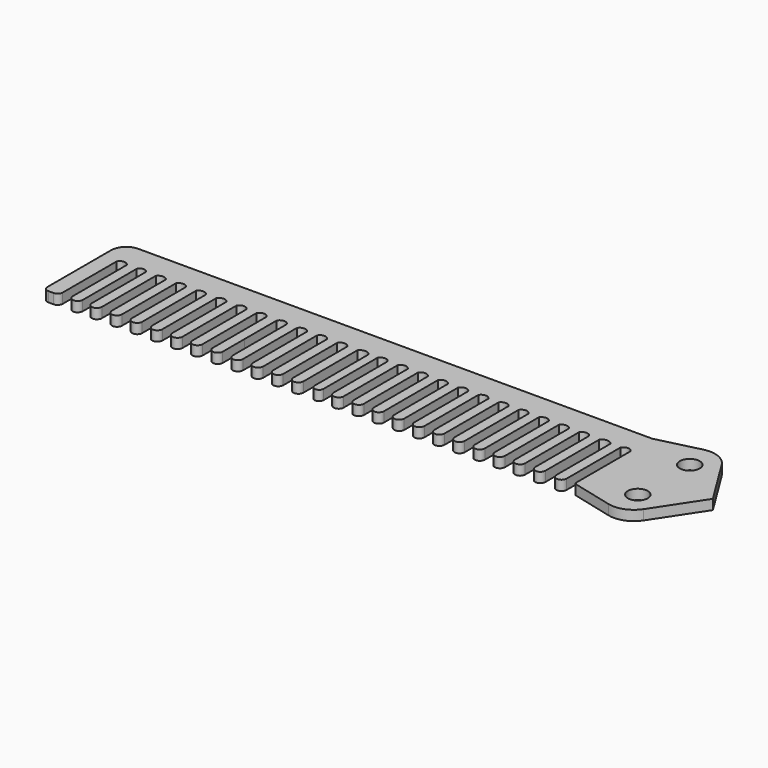
from build123d import *

# Parameters (mm, degrees)
F0_R     = 2
F1_DEPTH = 2


# Not quite as in the source:
# - a feature names something its author has since deleted; it is built from what else it names


with BuildPart() as f1:
    # F0 (on Top) → F1 (new body)
    with BuildSketch(Plane.XY):
        with BuildLine():
            ThreePointArc((-47.5321587284, -3.0349094544), (-47.2359537694, -3.7500114836), (-46.5208517402, -4.0462164426))
            Line((-46.5208517402, -4.0462164426), (-45.4874065769, -4.0462164426))
            ThreePointArc((-45.4874065769, -4.0462164426), (-44.7723045476, -3.7500114836), (-44.4760995886, -3.0349094544))
            Line((-44.4760995886, -3.0349094544), (-44.4760995886, 10.5057977874))
            ThreePointArc((-44.4760995886, 10.5057977874), (-43.4758616879, 11.1175826134), (-42.4756237872, 10.5057977874))
            Line((-42.4756237872, 10.5057977874), (-42.4756237872, -3.0349094544))
            Line((-42.4756237872, -3.0349094544), (-42.4756237872, -3.0449686175))
            ThreePointArc((-42.4756237872, -3.0449686175), (-41.464329306, -4.0512460242), (-40.4530348247, -3.0449686175))
            Line((-40.4530348247, -3.0449686175), (-40.4530348247, -3.0349094544))
            Line((-40.4530348247, -3.0349094544), (-40.4530348247, 2.3688513962))
            Line((-40.4530348247, 2.3688513962), (-40.4530348247, 10.5057977874))
            ThreePointArc((-40.4530348247, 10.5057977874), (-39.5547852119, 11.0928656343), (-38.6565355991, 10.5057977874))
            Line((-38.6565355991, 10.5057977874), (-38.6565355991, 2.3688513962))
            Line((-38.6565355991, 2.3688513962), (-38.6565355991, -3.0349094544))
            ThreePointArc((-38.6565355991, -3.0349094544), (-37.6453452622, -4.0308565278), (-36.6341549253, -3.0349094544))
            Line((-36.6341549253, -3.0349094544), (-36.6341549253, 2.3688513962))
            Line((-36.6341549253, 2.3688513962), (-36.6341549253, 10.5057977874))
            ThreePointArc((-36.6341549253, 10.5057977874), (-35.6227312857, 11.0363635), (-34.6113076461, 10.5057977874))
            Line((-34.6113076461, 10.5057977874), (-34.6113076461, 2.3688513962))
            Line((-34.6113076461, 2.3688513962), (-34.6113076461, -3.0349094544))
            ThreePointArc((-34.6113076461, -3.0349094544), (-33.6001581891, -4.0283670709), (-32.5890087321, -3.0349094544))
            Line((-32.5890087321, -3.0349094544), (-32.5890087321, 2.3688513962))
            Line((-32.5890087321, 2.3688513962), (-32.5890087321, 10.5057977874))
            ThreePointArc((-32.5890087321, 10.5057977874), (-31.5775442126, 11.0839798549), (-30.5660796932, 10.5057977874))
            Line((-30.5660796932, 10.5057977874), (-30.5660796932, 2.3688513962))
            Line((-30.5660796932, 2.3688513962), (-30.5660796932, -3.0349094544))
            ThreePointArc((-30.5660796932, -3.0349094544), (-29.5547727049, -4.0320483822), (-28.5434657167, -3.0349094544))
            Line((-28.5434657167, -3.0349094544), (-28.5434657167, 2.3688513962))
            Line((-28.5434657167, 2.3688513962), (-28.5434657167, 10.5057977874))
            ThreePointArc((-28.5434657167, 10.5057977874), (-27.5321587284, 11.0375669764), (-26.5208517402, 10.5057977874))
            Line((-26.5208517402, 10.5057977874), (-26.5208517402, 2.3688513962))
            Line((-26.5208517402, 2.3688513962), (-26.5208517402, -3.0349094544))
            ThreePointArc((-26.5208517402, -3.0349094544), (-25.5095447519, -4.0289367833), (-24.4982377637, -3.0349094544))
            Line((-24.4982377637, -3.0349094544), (-24.4982377637, 2.3688513962))
            Line((-24.4982377637, 2.3688513962), (-24.4982377637, 10.5057977874))
            ThreePointArc((-24.4982377637, 10.5057977874), (-23.4869307754, 11.0979693494), (-22.4756237872, 10.5057977874))
            Line((-22.4756237872, 10.5057977874), (-22.4756237872, 2.3688513962))
            Line((-22.4756237872, 2.3688513962), (-22.4756237872, -3.0349094544))
            ThreePointArc((-22.4756237872, -3.0349094544), (-21.464316799, -4.0179106089), (-20.4530098107, -3.0349094544))
            Line((-20.4530098107, -3.0349094544), (-20.4530098107, 2.3688513962))
            Line((-20.4530098107, 2.3688513962), (-20.4530098107, 10.5057977874))
            ThreePointArc((-20.4530098107, 10.5057977874), (-19.4417028225, 11.112544636), (-18.4303958342, 10.5057977874))
            Line((-18.4303958342, 10.5057977874), (-18.4303958342, 2.3688513962))
            Line((-18.4303958342, 2.3688513962), (-18.4303958342, -3.0349094544))
            ThreePointArc((-18.4303958342, -3.0349094544), (-17.419088846, -4.0462164426), (-16.4077818577, -3.0349094544))
            Line((-16.4077818577, -3.0349094544), (-16.4077818577, 2.3688513962))
            Line((-16.4077818577, 2.3688513962), (-16.4077818577, 10.5057977874))
            ThreePointArc((-16.4077818577, 10.5057977874), (-15.3964748695, 11.0913376707), (-14.3851678813, 10.5057977874))
            Line((-14.3851678813, 10.5057977874), (-14.3851678812, 2.3688513962))
            Line((-14.3851678812, 2.3688513962), (-14.3851678812, -3.0349094544))
            ThreePointArc((-14.3851678812, -3.0349094544), (-13.373860893, -4.0324857923), (-12.3625539048, -3.0349094544))
            Line((-12.3625539048, -3.0349094544), (-12.3625539048, 2.3688513962))
            Line((-12.3625539047, 2.3688513962), (-12.3625539048, 10.5057977874))
            ThreePointArc((-12.3625539048, 10.5057977874), (-11.3512469165, 11.1038299062), (-10.3399399283, 10.5057977874))
            Line((-10.3399399283, 10.5057977874), (-10.3399399283, 2.3688513962))
            Line((-10.3399399283, 2.3688513962), (-10.3399399283, -3.0349094544))
            ThreePointArc((-10.3399399283, -3.0349094544), (-9.32863294, -4.0336439564), (-8.3173259518, -3.0349094544))
            Line((-8.3173259518, -3.0349094544), (-8.3173259518, 2.3688513962))
            Line((-8.3173259518, 2.3688513962), (-8.3173259518, 10.5057977874))
            ThreePointArc((-8.3173259518, 10.5057977874), (-7.3060189635, 11.1037566218), (-6.2947119753, 10.5057977874))
            Line((-6.2947119753, 10.5057977874), (-6.2947119753, 2.3688513962))
            Line((-6.2947119753, 2.3688513962), (-6.2947119753, -3.0349094544))
            ThreePointArc((-6.2947119753, -3.0349094544), (-5.283404987, -4.0328236585), (-4.2720979988, -3.0349094544))
            Line((-4.2720979988, -3.0349094544), (-4.2720979988, 2.3688513962))
            Line((-4.2720979988, 2.3688513962), (-4.2720979988, 10.5057977874))
            ThreePointArc((-4.2720979988, 10.5057977874), (-3.2607910105, 11.1182503387), (-2.2494840223, 10.5057977874))
            Line((-2.2494840223, 10.5057977874), (-2.2494840223, 2.3688513962))
            Line((-2.2494840223, 2.3688513962), (-2.2494840223, -3.0349094544))
            ThreePointArc((-2.2494840223, -3.0349094544), (-1.2381770341, -4.0279358965), (-0.2268700458, -3.0349094544))
            Line((-0.2268700458, -3.0349094544), (-0.2268700458, 2.3688513962))
            Line((-0.2268700458, 2.3688513962), (-0.2268700458, 10.5057977874))
            ThreePointArc((-0.2268700458, 10.5057977874), (0.7844369424, 11.1117892762), (1.7957439307, 10.5057977874))
            Line((1.7957439307, 10.5057977874), (1.7957439307, 2.3688513962))
            Line((1.7957439307, 2.3688513962), (1.7957439307, -3.0349094544))
            ThreePointArc((1.7957439307, -3.0349094544), (2.8070509189, -4.0231444656), (3.8183579072, -3.0349094544))
            Line((3.8183579072, -3.0349094544), (3.8183579072, 2.3688513962))
            Line((3.8183579072, 2.3688513962), (3.8183579072, 10.5057977874))
            ThreePointArc((3.8183579072, 10.5057977874), (4.9481016159, 11.1006888991), (6.0778453246, 10.5057977874))
            Line((6.0778453246, 10.5057977874), (6.0778453246, 2.3688513962))
            Line((6.0778453246, 2.3688513962), (6.0778453246, -3.0349094544))
            ThreePointArc((6.0778453246, -3.0349094544), (6.9707155924, -3.9277797221), (7.8635858601, -3.0349094544))
            Line((7.8635858601, -3.0349094544), (7.8635858601, 2.3688513962))
            Line((7.8635858601, 2.3688513962), (7.8635858601, 10.5057977874))
            ThreePointArc((7.8635858601, 10.5057977874), (8.8748928484, 11.1003156957), (9.8861998366, 10.5057977874))
            Line((9.8861998366, 10.5057977874), (9.8861998366, 2.3688513962))
            Line((9.8861998366, 2.3688513962), (9.8861998366, -3.0349094544))
            ThreePointArc((9.8861998366, -3.0349094544), (10.8975068249, -4.0462164426), (11.9088138131, -3.0349094544))
            Line((11.9088138131, -3.0349094544), (11.9088138131, 2.3688513962))
            Line((11.9088138131, 2.3688513962), (11.9088138131, 10.5057977874))
            ThreePointArc((11.9088138131, 10.5057977874), (12.9201208014, 11.1003953408), (13.9314277896, 10.5057977874))
            Line((13.9314277896, 10.5057977874), (13.9314277896, 2.3688513962))
            Line((13.9314277896, 2.3688513962), (13.9314277896, -3.0349094544))
            ThreePointArc((13.9314277896, -3.0349094544), (14.9427347779, -4.0462164426), (15.9540417661, -3.0349094544))
            Line((15.9540417661, -3.0349094544), (15.9540417661, 2.3688513962))
            Line((15.9540417661, 2.3688513962), (15.9540417661, 10.5057977874))
            ThreePointArc((15.9540417661, 10.5057977874), (16.9653487543, 11.1012729968), (17.9766557426, 10.5057977874))
            Line((17.9766557426, 10.5057977874), (17.9766557426, -3.0349094544))
            Line((17.9766557426, -3.0349094544), (17.9766557426, -3.0600128507))
            ThreePointArc((17.9766557426, -3.0600128507), (18.987884836, -4.0587681408), (19.9991139294, -3.0600128507))
            Line((19.9991139294, -3.0600128507), (19.9991139294, -3.0349094544))
            Line((19.9991139294, -3.0349094544), (19.9991139294, 2.3688513962))
            Line((19.9991139294, 2.3688513962), (19.9991139294, 10.5057977874))
            ThreePointArc((19.9991139294, 10.5057977874), (21.0104988125, 11.0625593301), (22.0218836956, 10.5057977874))
            Line((22.0218836956, 10.5057977874), (22.0218836956, 2.3688513962))
            Line((22.0218836956, 2.3688513962), (22.0218836956, -3.0349094544))
            ThreePointArc((22.0218836956, -3.0349094544), (23.0331906838, -4.0270898738), (24.0444976721, -3.0349094544))
            Line((24.0444976721, -3.0349094544), (24.0444976721, 2.3688513962))
            Line((24.0444976721, 2.3688513962), (24.0444976721, 10.5057977874))
            ThreePointArc((24.0444976721, 10.5057977874), (25.0558046603, 11.1004906415), (26.0671116486, 10.5057977874))
            Line((26.0671116486, 10.5057977874), (26.0671116486, 2.3688513962))
            Line((26.0671116486, 2.3688513962), (26.0671116486, -3.0349094544))
            ThreePointArc((26.0671116486, -3.0349094544), (27.0784186368, -4.0282444578), (28.089725625, -3.0349094544))
            Line((28.089725625, -3.0349094544), (28.089725625, 2.3688513962))
            Line((28.089725625, 2.3688513962), (28.089725625, 10.5057977874))
            ThreePointArc((28.089725625, 10.5057977874), (29.1010326133, 11.1005861122), (30.1123396015, 10.5057977874))
            Line((30.1123396015, 10.5057977874), (30.1123396015, 2.3688513962))
            Line((30.1123396015, 2.3688513962), (30.1123396015, -3.0349094544))
            ThreePointArc((30.1123396015, -3.0349094544), (31.1236465898, -4.0401241658), (32.134953578, -3.0349094544))
            Line((32.134953578, -3.0349094544), (32.134953578, 2.3688513962))
            Line((32.134953578, 2.3688513962), (32.134953578, 10.5057977874))
            ThreePointArc((32.134953578, 10.5057977874), (33.1462605663, 11.0805944093), (34.1575675545, 10.5057977874))
            Line((34.1575675545, 10.5057977874), (34.1575675545, 2.3688513962))
            Line((34.1575675545, 2.3688513962), (34.1575675545, -3.0349094544))
            ThreePointArc((34.1575675545, -3.0349094544), (35.1688745428, -4.0284589293), (36.180181531, -3.0349094544))
            Line((36.180181531, -3.0349094544), (36.180181531, 2.3688513962))
            Line((36.180181531, 2.3688513962), (36.180181531, 10.5057977874))
            ThreePointArc((36.180181531, 10.5057977874), (37.1914885192, 11.0806196167), (38.2027955075, 10.5057977874))
            Line((38.2027955075, 10.5057977874), (38.2027955075, 2.3688513962))
            Line((38.2027955075, 2.3688513962), (38.2027955075, -3.0349094544))
            ThreePointArc((38.2027955075, -3.0349094544), (39.2141024957, -4.0246480782), (40.225409484, -3.0349094544))
            Line((40.225409484, -3.0349094544), (40.225409484, 2.3688513962))
            Line((40.225409484, 2.3688513962), (40.225409484, 10.5057977874))
            ThreePointArc((40.225409484, 10.5057977874), (41.2367164722, 11.0799992786), (42.2480234605, 10.5057977874))
            Line((42.2480234605, 10.5057977874), (42.2480234605, 2.3688513962))
            Line((42.2480234605, 2.3688513962), (42.2480234605, -3.0349094544))
            ThreePointArc((42.2480234605, -3.0349094544), (43.2593304487, -4.0462164426), (44.270637437, -3.0349094544))
            Line((44.270637437, -3.0349094544), (44.270637437, 2.3688513962))
            Line((44.270637437, 2.3688513962), (44.270637437, 10.5057977874))
            ThreePointArc((44.270637437, 10.5057977874), (45.2819444252, 11.0763000676), (46.2932514135, 10.5057977874))
            Line((46.2932514135, 10.5057977874), (46.2932514135, 2.3688513962))
            Line((46.2932514135, 2.3688513962), (46.2932514135, -3.0349094544))
            ThreePointArc((46.2932514135, -3.0349094544), (47.3045584017, -4.0362897846), (48.3158653899, -3.0349094544))
            Line((48.3158653899, -3.0349094544), (48.3158653899, 2.3688513962))
            Line((48.3158653899, 2.3688513962), (48.3158653899, 10.5057977874))
            ThreePointArc((48.3158653899, 10.5057977874), (49.3271723782, 11.0768378201), (50.3384793664, 10.5057977874))
            Line((50.3384793664, 10.5057977874), (50.3384793664, 2.3688513962))
            Line((50.3384793664, 2.3688513962), (50.3384793664, -3.0349094544))
            ThreePointArc((50.3384793664, -3.0349094544), (51.3497863547, -4.0273604844), (52.3610933429, -3.0349094544))
            Line((52.3610933429, -3.0349094544), (52.3610933429, 2.3688513962))
            Line((52.3610933429, 2.3688513962), (52.3610933429, 10.5057977874))
            ThreePointArc((52.3610933429, 10.5057977874), (53.4851541573, 11.0994017223), (54.6092149717, 10.5057977874))
            Line((54.6092149717, 10.5057977874), (54.6092149717, 2.3688513962))
            Line((54.6092149717, 2.3688513962), (54.6092149717, -3.0349094544))
            ThreePointArc((54.6092149717, -3.0349094544), (55.6205026048, -4.039959639), (56.6317902379, -3.0349094544))
            Line((56.6317902379, -3.0349094544), (56.6317902379, 10.5057977874))
            ThreePointArc((56.6317902379, 10.5057977874), (57.6430972262, 11.0968589506), (58.6544042144, 10.5057977874))
            Line((58.6544042144, 10.5057977874), (58.6544042144, -3.183207694))
            ThreePointArc((58.6544042144, -3.183207694), (58.6957151001, -3.3833861096), (58.8128977225, -3.5508561677))
            Line((58.8128977225, -3.5508561677), (67.1425286707, -5.6492492557))
            ThreePointArc((67.1425286707, -5.6492492557), (70.1745553832, -5.4613941054), (72.5382215144, -3.553107449))
            Line((72.5382215144, -3.553107449), (78.7976136626, 5.9399087982))
            ThreePointArc((78.7976136626, 5.9399087982), (78.7234830832, 6.1327797263), (78.5951017421, 6.2946833056))
            Line((78.5951017421, 6.2946833056), (72.6648820615, 15.8458770867))
            ThreePointArc((72.6648820615, 15.8458770867), (70.3034587252, 17.8389512741), (67.2215312081, 18.0634232527))
            Line((67.2215312081, 18.0634232527), (58.6544042144, 15.9537835574))
            Line((58.6544042144, 15.9537835574), (-44.4982377637, 15.9537835574))
            ThreePointArc((-44.4982377637, 15.9537835574), (-46.6435438514, 15.0651686804), (-47.5321587284, 12.9198625927))
            Line((-47.5321587284, 12.9198625927), (-47.5321587284, -3.0349094544))
        make_face()
        with Locations((68.7303330245, -0.2896678891)):
            Circle(F0_R, mode=Mode.SUBTRACT)
        with Locations((68.7701961271, 12.7037232041)):
            Circle(F0_R, mode=Mode.SUBTRACT)
    extrude(amount=F1_DEPTH)


solid = f1.part
